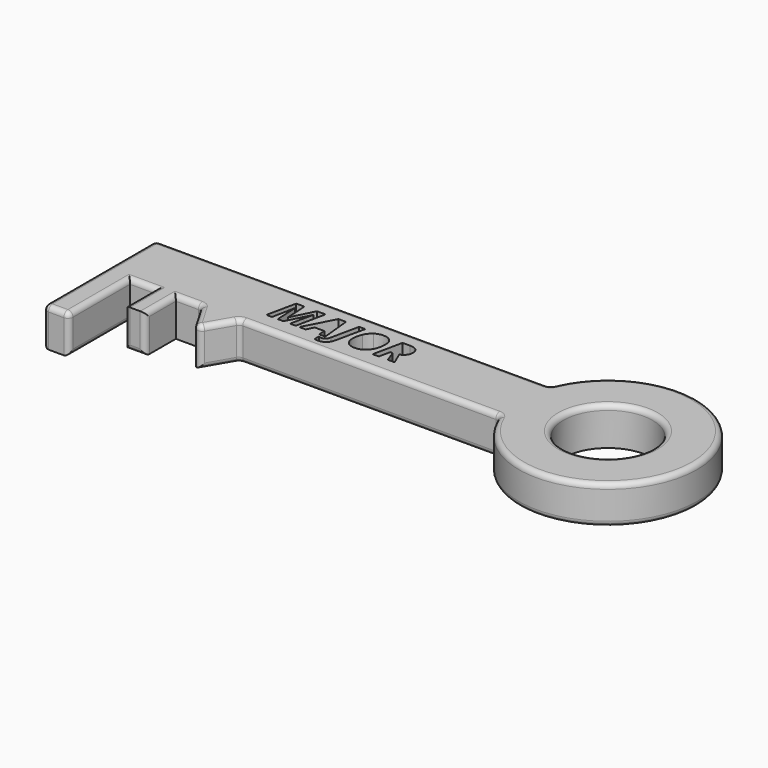
from build123d import *

# Parameters (mm, degrees)
F0_R     = 17.5
F1_DEPTH = 15
F2_R     = 2


with BuildPart() as f1:
    # F0 (on Top) → F1 (new body)
    with BuildSketch(Plane.XY):
        with BuildLine():
            ThreePointArc((14.5522479275, -12.5), (82.2439900041, 0), (14.5522479275, 12.5))
            Line((14.5522479275, 12.5), (-140.4477520725, 12.5))
            Line((-140.4477520725, 12.5), (-140.4477520725, -12.5))
            Line((-140.4477520725, -12.5), (-140.4477520725, -42.5))
            Line((-140.4477520725, -42.5), (-130.4477520725, -42.5))
            Line((-130.4477520725, -42.5), (-130.4477520725, -12.5))
            Line((-130.4477520725, -12.5), (-120.4477520725, -12.5))
            Line((-120.4477520725, -12.5), (-120.4477520725, -27.5))
            Line((-120.4477520725, -27.5), (-112.4477520725, -27.5))
            Line((-112.4477520725, -27.5), (-112.4477520725, -12.5))
            Line((-112.4477520725, -12.5), (-102.4477520725, -12.5))
            Line((-102.4477520725, -12.5), (-94.8704325514, -25.4454327419))
            Line((-94.8704325514, -25.4454327419), (-87.2931130304, -12.5))
            Line((-87.2931130304, -12.5), (14.5522479275, -12.5))
        make_face()
        with BuildLine():
            Line((-76.5016191468, -2.3224616444), (-76.4686113325, -2.3224616444))
            Line((-76.4686113325, -2.3224616444), (-72.0963454781, 6.3509763107))
            Line((-72.0963454781, 6.3509763107), (-68.739704677, 6.3509763107))
            Line((-68.739704677, 6.3509763107), (-71.1924391807, -5.2500008605))
            Line((-71.1924391807, -5.2500008605), (-73.4141189848, -5.2500008605))
            Line((-73.4141189848, -5.2500008605), (-72.2639236119, 0.2419916151))
            add(Edge.make_bspline(
                [(-72.2639236119, 0.2419916151), (-71.8424392148, 2.1996089054), (-71.4311110682, 3.7408199237)],
                knots=[0, 0, 0, 1, 1, 1], degree=2))
            Line((-71.4311110682, 3.7408199237), (-71.4691970077, 3.7408199237))
            Line((-71.4691970077, 3.7408199237), (-75.9861894322, -5.2500008605))
            Line((-75.9861894322, -5.2500008605), (-78.2154864242, -5.2500008605))
            Line((-78.2154864242, -5.2500008605), (-78.6979083245, 3.7408199237))
            Line((-78.6979083245, 3.7408199237), (-78.7309161387, 3.7408199237))
            add(Edge.make_bspline(
                [(-78.7309161387, 3.7408199237), (-78.8172442683, 3.0425776996), (-79.0317950608, 1.9076167025)],
                knots=[0, 0, 0, 1, 1, 1], degree=2))
            add(Edge.make_bspline(
                [(-79.0317950608, 1.9076167025), (-79.2463458533, 0.7726557055), (-80.5158771699, -5.2500008605)],
                knots=[0, 0, 0, 1, 1, 1], degree=2))
            Line((-80.5158771699, -5.2500008605), (-82.6969319718, -5.2500008605))
            Line((-82.6969319718, -5.2500008605), (-80.2467365308, 6.3509763107))
            Line((-80.2467365308, 6.3509763107), (-77.039900425, 6.3509763107))
            Line((-77.039900425, 6.3509763107), (-76.5016191468, -2.3224616444))
        make_face(mode=Mode.SUBTRACT)
        Polygon((-61.9502511957, -5.2500008605), (-62.1406808932, -2.4875007156), (-65.8934154651, -2.4875007156), (-67.2568920992, -5.2500008605), (-69.7959547324, -5.2500008605), (-63.7199778511, 6.3992185007), (-60.7594308207, 6.3992185007), (-59.5940010721, -5.2500008605), align=None, mode=Mode.SUBTRACT)
        with BuildLine():
            add(Edge.make_bspline(
                [(-56.9381415577, -7.773829118), (-57.9182197341, -8.6625010396), (-59.6879463895, -8.6625010396)],
                knots=[0, 0, 0, 1, 1, 1], degree=2))
            add(Edge.make_bspline(
                [(-59.6879463895, -8.6625010396), (-60.4344308037, -8.6625010396), (-61.1707589673, -8.4466807158)],
                knots=[0, 0, 0, 1, 1, 1], degree=2))
            Line((-61.1707589673, -8.4466807158), (-61.1707589673, -6.4408212355))
            add(Edge.make_bspline(
                [(-61.1707589673, -6.4408212355), (-60.4725167432, -6.5982431188), (-59.8707588991, -6.5982431188)],
                knots=[0, 0, 0, 1, 1, 1], degree=2))
            add(Edge.make_bspline(
                [(-59.8707588991, -6.5982431188), (-59.0836494828, -6.5982431188), (-58.5961494572, -6.1183602811)],
                knots=[0, 0, 0, 1, 1, 1], degree=2))
            add(Edge.make_bspline(
                [(-58.5961494572, -6.1183602811), (-58.1086494316, -5.6384774434), (-57.8852119199, -4.6000008264)],
                knots=[0, 0, 0, 1, 1, 1], degree=2))
            Line((-57.8852119199, -4.6000008264), (-55.5619696105, 6.3509763107))
            Line((-55.5619696105, 6.3509763107), (-53.142242921, 6.3509763107))
            Line((-53.142242921, 6.3509763107), (-55.5467352347, -4.9402352193))
            add(Edge.make_bspline(
                [(-55.5467352347, -4.9402352193), (-55.9580633813, -6.8851571963), (-56.9381415577, -7.773829118)],
                knots=[0, 0, 0, 1, 1, 1], degree=2))
        make_face(mode=Mode.SUBTRACT)
        with BuildLine():
            add(Edge.make_bspline(
                [(-42.9847228568, 5.3912106353), (-41.8738829548, 4.2486324504), (-41.8738829548, 2.1919917175)],
                knots=[0, 0, 0, 1, 1, 1], degree=2))
            add(Edge.make_bspline(
                [(-41.8738829548, 2.1919917175), (-41.8738829548, -0.0525396503), (-42.6597228397, -1.8260748996)],
                knots=[0, 0, 0, 1, 1, 1], degree=2))
            add(Edge.make_bspline(
                [(-42.6597228397, -1.8260748996), (-43.4455627247, -3.5996101489), (-44.8103088901, -4.5047859777)],
                knots=[0, 0, 0, 1, 1, 1], degree=2))
            add(Edge.make_bspline(
                [(-44.8103088901, -4.5047859777), (-46.1750550555, -5.4099618064), (-47.9523988987, -5.4099618064)],
                knots=[0, 0, 0, 1, 1, 1], degree=2))
            add(Edge.make_bspline(
                [(-47.9523988987, -5.4099618064), (-49.9836490053, -5.4099618064), (-51.1224185963, -4.2394539325)],
                knots=[0, 0, 0, 1, 1, 1], degree=2))
            add(Edge.make_bspline(
                [(-51.1224185963, -4.2394539325), (-52.2611881873, -3.0689460586), (-52.2611881873, -0.989453762)],
                knots=[0, 0, 0, 1, 1, 1], degree=2))
            add(Edge.make_bspline(
                [(-52.2611881873, -0.989453762), (-52.2611881873, 1.1128900983), (-51.4753483023, 2.8788081597)],
                knots=[0, 0, 0, 1, 1, 1], degree=2))
            add(Edge.make_bspline(
                [(-51.4753483023, 2.8788081597), (-50.6895084173, 4.6447262212), (-49.3082583449, 5.5892575207)],
                knots=[0, 0, 0, 1, 1, 1], degree=2))
            add(Edge.make_bspline(
                [(-49.3082583449, 5.5892575207), (-47.9270082724, 6.5337888203), (-46.1191956775, 6.5337888203)],
                knots=[0, 0, 0, 1, 1, 1], degree=2))
            add(Edge.make_bspline(
                [(-46.1191956775, 6.5337888203), (-44.0955627588, 6.5337888203), (-42.9847228568, 5.3912106353)],
                knots=[0, 0, 0, 1, 1, 1], degree=2))
        make_face(mode=Mode.SUBTRACT)
        with BuildLine():
            Line((-36.6434139303, -0.7990240645), (-37.5879452299, -0.7990240645))
            Line((-37.5879452299, -0.7990240645), (-38.5324765294, -5.2500008605))
            Line((-38.5324765294, -5.2500008605), (-40.9522032189, -5.2500008605))
            Line((-40.9522032189, -5.2500008605), (-38.5020077778, 6.3509763107))
            Line((-38.5020077778, 6.3509763107), (-35.6531795033, 6.3509763107))
            add(Edge.make_bspline(
                [(-35.6531795033, 6.3509763107), (-33.7717340921, 6.3509763107), (-32.8272027926, 5.5410153307)],
                knots=[0, 0, 0, 1, 1, 1], degree=2))
            add(Edge.make_bspline(
                [(-32.8272027926, 5.5410153307), (-31.882671493, 4.7310543507), (-31.882671493, 3.1695308313)],
                knots=[0, 0, 0, 1, 1, 1], degree=2))
            add(Edge.make_bspline(
                [(-31.882671493, 3.1695308313), (-31.882671493, 1.9152338904), (-32.5415582463, 1.015136187)],
                knots=[0, 0, 0, 1, 1, 1], degree=2))
            add(Edge.make_bspline(
                [(-32.5415582463, 1.015136187), (-33.2004449996, 0.1150384835), (-34.4395075647, -0.3216802894)],
                knots=[0, 0, 0, 1, 1, 1], degree=2))
            Line((-34.4395075647, -0.3216802894), (-32.3676324559, -5.2500008605))
            Line((-32.3676324559, -5.2500008605), (-35.0031794692, -5.2500008605))
            Line((-35.0031794692, -5.2500008605), (-36.6434139303, -0.7990240645))
        make_face(mode=Mode.SUBTRACT)
        with Locations((47.2439900041, 0)):
            Circle(F0_R, mode=Mode.SUBTRACT)
    extrude(amount=F1_DEPTH)

    # F2
    f2_edges = [f1.edges().sort_by_distance(p)[0] for p in [
        (-62.947752, 12.5, 15),
        (82.24399, 0, 15),
        (-36.370433, -12.5, 15),
        (29.74399, 0, 15),
        (-91.081773, -18.972716, 15),
        (-98.659092, -18.972716, 15),
        (-107.447752, -12.5, 15),
        (-112.447752, -20, 15),
        (-120.447752, -20, 15),
        (-130.447752, -27.5, 15),
        (-140.447752, -15, 15),
        (-135.447752, -42.5, 15),
        (-62.947752, 12.5, 0),
        (-140.447752, 12.5, 7.5),
        (-140.447752, -15, 0),
        (-140.447752, -42.5, 7.5),
        (82.24399, 0, 0),
        (-130.447752, -27.5, 0),
        (-116.447752, -27.5, 0),
        (-130.447752, -42.5, 7.5),
        (-120.447752, -27.5, 7.5),
        (-102.447752, -12.5, 7.5),
        (-94.870433, -25.445433, 7.5),
        (-87.293113, -12.5, 7.5),
        (-112.447752, -27.5, 7.5),
        (14.552248, 12.5, 7.5),
        (14.552248, -12.5, 7.5),
        (-36.370433, -12.5, 0),
        (-125.447752, -12.5, 15),
        (-91.081773, -18.972716, 0),
    ]]
    fillet(f2_edges, radius=F2_R)


solid = f1.part
